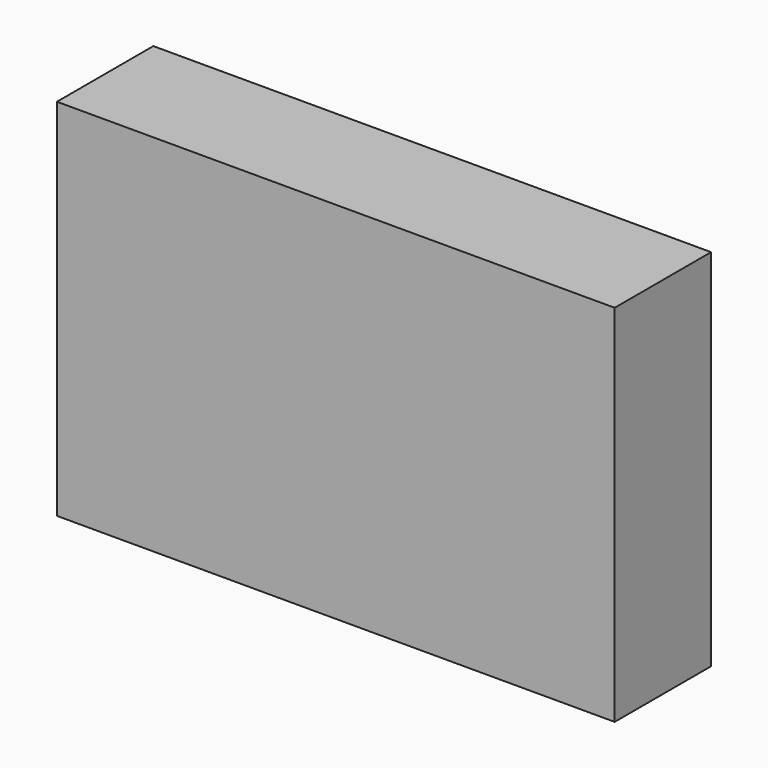
from build123d import *

# Parameters (mm, degrees)
F0_W     = 70.5431774259
F0_H     = 46.1126379669
F1_DEPTH = 15.24


# Not quite as in the source:
# - the program builds the solid bodies; features that only make, move or delete a surface that nothing else refers to are left out


with BuildPart() as f1:
    # F0 (on Front) → F1 (new body)
    with BuildSketch(Plane.XZ):
        Rectangle(F0_W, F0_H)
    extrude(amount=F1_DEPTH)


solid = f1.part
